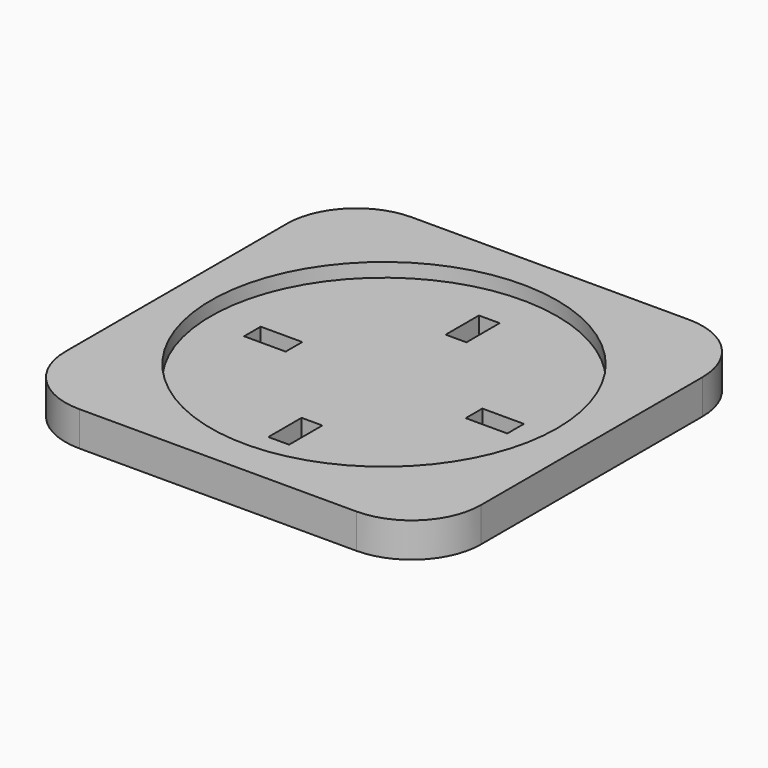
from build123d import *

# Parameters (mm, degrees)
F0_W            = 60
F0_H            = 60
F1_DEPTH        = 5
F2_R            = 25
F3_DEPTH        = 2
F4_R            = 10
F5_W            = 3
F5_H            = 6
F6_DEPTH        = 25
F6_COPIES_COUNT = 4


# Not quite as in the source:
# - a pattern or mirror of a feature is missing from the dataset's text; its kind, count and spacing are read off the source's solid
# - a feature names something its author has since deleted; it is built from what else it names


with BuildPart() as f1:
    # F0 (on Top) → F1 (new body)
    with BuildSketch(Plane.XY):
        Rectangle(F0_W, F0_H)
    extrude(amount=F1_DEPTH)

    # F2 (on face) → F3 (cut)
    with BuildSketch(Plane.XY.offset(5)):
        Circle(F2_R)
    extrude(amount=-F3_DEPTH, mode=Mode.SUBTRACT)

    # F4
    f4_edges = [f1.edges().sort_by_distance(p)[0] for p in [
        (-30, -30, 2.5),
        (30, -30, 2.5),
        (30, 30, 2.5),
        (-30, 30, 2.5),
    ]]
    fillet(f4_edges, radius=F4_R)

    # F5 (on face) → F6 (cut)
    with BuildSketch(Plane.XY.offset(3)):
        with Locations((0, 16)):
            Rectangle(F5_W, F5_H)
    f6 = extrude(amount=-F6_DEPTH, mode=Mode.SUBTRACT)

    # F6_copies: F6 ×4 about axis
    f6_copies_axis = Axis((0, 0, 0), (0, 0, 1))
    for i in range(1, F6_COPIES_COUNT):
        add(f6.rotate(f6_copies_axis, i * 360 / F6_COPIES_COUNT), mode=Mode.SUBTRACT)


solid = f1.part
